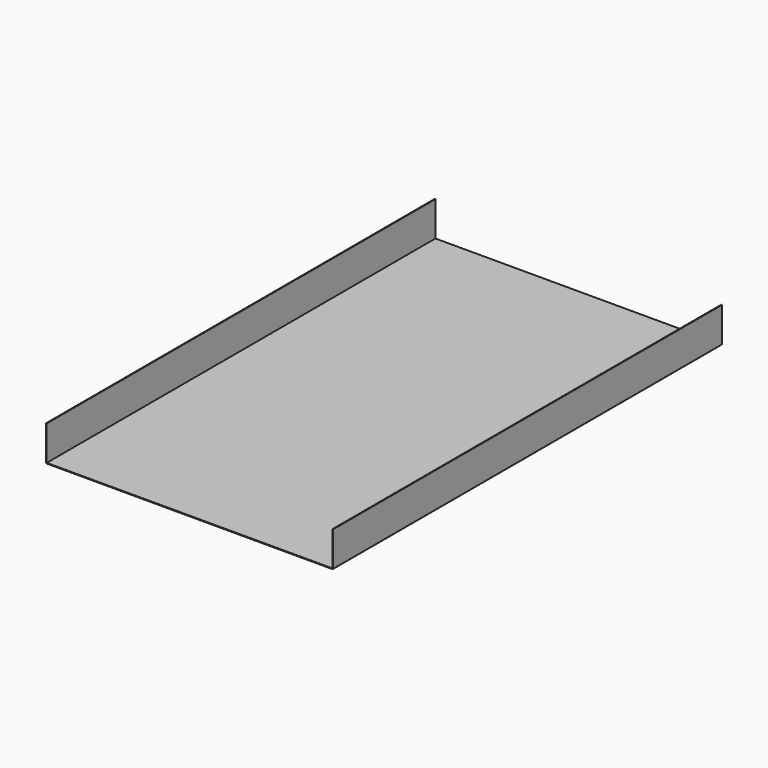
from build123d import *

# Parameters (mm, degrees)
F0_W        = 650
F0_H        = 1100
F1_DEPTH    = 1.5
F2_W        = 1100
F2_H        = 78.5
F3_DEPTH    = 1.5
F4_T1_DEPTH = 1109.6824583655
F5_W        = 1100
F5_H        = 78.5
F6_DEPTH    = 1.5
F7_R        = 2


# Not quite as in the source:
# - a fillet or chamfer that OpenCascade refuses, or shapes differently, is made with other operations: its cross-section is extruded or revolved along the edge and cut away or added


with BuildPart() as f1:
    # F0 (on Top) → F1 (new body)
    with BuildSketch(Plane.XY):
        with Locations((16.3806613057, 550)):
            Rectangle(F0_W, F0_H)
    extrude(amount=F1_DEPTH)

    # F4: fillet of radius 2 on 1 edges, made by hand

    # F4_s2 → F4_t1 (cut)
    with BuildSketch(Plane.XZ.offset(-1104.8412291828)):
        with BuildLine():
            ThreePointArc((-308.6193386943, 1.5), (-307.9075918926, 0.4188611699), (-306.6828470212, 0))
            Line((-306.6828470212, 0), (-308.6193386943, 0))
            Line((-308.6193386943, 0), (-308.6193386943, 1.5))
        make_face()
    extrude(amount=F4_T1_DEPTH, mode=Mode.SUBTRACT)

    # F5 (on face) → F6 (join)
    with BuildSketch(Plane.YZ.offset(341.3806613057)):
        with Locations((550, 40.75)):
            Rectangle(F5_W, F5_H)
    extrude(amount=-F6_DEPTH)

    # F7
    f7_edges = [f1.edges().sort_by_distance(p)[0] for p in [
        (341.380661, 550, 0),
    ]]
    fillet(f7_edges, radius=F7_R)


with BuildPart() as f3:
    # F2 (on face) → F3 (new body)
    with BuildSketch(Plane(origin=(-308.6193386943, 0, 0), x_dir=(0, -1, 0), z_dir=(-1, 0, 0))):
        with Locations((-550, 40.75)):
            Rectangle(F2_W, F2_H)
    extrude(amount=-F3_DEPTH)


solid = Compound([f1.part, f3.part])
